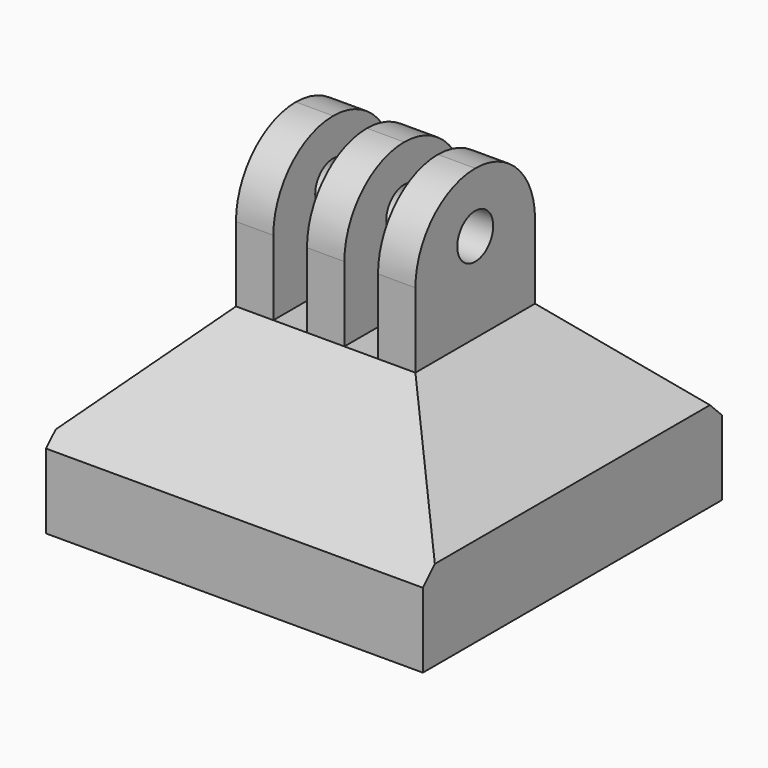
from build123d import *

# Parameters (mm, degrees)
F1_DEPTH     = 10
F2_R         = 4.99999
F3_W         = 7.5
F3_H         = 5
F3_W_2       = 10
F4_DEPTH     = 25.2
F5_T1_DEPTH  = 12
F5_T6_DEPTH  = 10
F5_T11_DEPTH = 10
F5_T17_DEPTH = 29.2876224097
F5_T23_DEPTH = 31.2876224097
F5_T31_DEPTH = 29.2876224097
F5_T37_DEPTH = 31.2876224097
F5_T45_DEPTH = 29.2876224097
F5_T51_DEPTH = 31.2876224097
F5_T59_DEPTH = 31.2876224097
F5_T64_DEPTH = 29.2876224097
F6_R         = 1.5
F7_DEPTH     = 25


# Not quite as in the source:
# - a fillet or chamfer that OpenCascade refuses, or shapes differently, is made with other operations: its cross-section is extruded or revolved along the edge and cut away or added
# - a fillet or chamfer is up to 0.001 mm smaller than in the source, because OpenCascade refuses the exact size


with BuildPart() as f1:
    # F0 (on Front) → F1 (new body)
    with BuildSketch(Plane.XZ):
        Polygon((12.5, -2.5), (12.5, 2.5), (6, 2.5), (-6, 2.5), (-12.5, 2.5), (-12.5, -2.5), align=None)
        Polygon((-6, 2.5), (6, 2.5), (6, 10), (6, 20), (3.5, 20), (3.5, 10), (1.25, 10), (1.25, 20), (0, 20), (-1.25, 20), (-1.25, 10), (-3.5, 10), (-3.5, 20), (-6, 20), (-6, 10), align=None)
    extrude(amount=F1_DEPTH)

    # F2 (radius 5 in the source; OpenCascade refuses exactly that, so slightly less here)
    f2_edges = [f1.edges().sort_by_distance(p)[0] for p in [
        (-4.75, 0, 20),
        (0, 0, 20),
        (4.75, 0, 20),
        (-4.75, -10, 20),
        (0, -10, 20),
        (4.75, -10, 20),
    ]]
    fillet(f2_edges, radius=F2_R)

    # F3 (on face) → F4 (join)
    with BuildSketch(Plane.YZ.offset(12.5)):
        with Locations((-13.75, 0)):
            Rectangle(F3_W, F3_H)
        with Locations((3.75, 0)):
            Rectangle(F3_W, F3_H)
        with Locations((-5, 0)):
            Rectangle(F3_W_2, F3_H)
    extrude(amount=-F4_DEPTH)

    # F5: chamfer of 7.5 on 4 edges, made by hand

    # F5_s2 → F5_t1 (join)
    with BuildSketch(Plane.YZ.offset(-6)):
        Polygon((-17.5, 2.5), (-10, 10), (-10, 2.5), align=None)
        Polygon((7.5, 2.5), (0, 10), (0, 2.5), align=None)
    extrude(amount=F5_T1_DEPTH)


with BuildPart() as f5_tool4:
    # F5_s5 → F5_t6 (new body)
    with BuildSketch(Plane.XZ):
        Polygon((6, 10), (13.5, 2.5), (6, 2.5), align=None)
    extrude(amount=F5_T6_DEPTH)

    split(bisect_by=Plane.YZ.offset(12.5), keep=Keep.BOTTOM)


with BuildPart() as f1_1:
    add(f1.part)

    # F5_t3: union F5_tool4
    add(f5_tool4.part)


with BuildPart() as f5_tool9:
    # F5_s10 → F5_t11 (new body)
    with BuildSketch(Plane.XZ):
        Polygon((-13.5, 2.5), (-6, 10), (-6, 2.5), align=None)
    extrude(amount=F5_T11_DEPTH)

    split(bisect_by=Plane.YZ.offset(-12.7), keep=Keep.TOP)


with BuildPart() as f1_2:
    add(f1_1.part)

    # F5_t8: union F5_tool9
    add(f5_tool9.part)


with BuildPart() as f5_tool15:
    # F5_s16 → F5_t17 (new body)
    with BuildSketch(Plane.XZ):
        Polygon((6, 10), (13.5, 2.5), (6, 2.5), align=None)
    extrude(amount=F5_T17_DEPTH)

    split(bisect_by=Plane.XZ.offset(17.5), keep=Keep.BOTTOM)

    split(bisect_by=Plane.YZ.offset(12.5), keep=Keep.BOTTOM)

    split(bisect_by=Plane.XZ.offset(10), keep=Keep.TOP)


with BuildPart() as f5_tool21:
    # F5_s22 → F5_t23 (new body)
    with BuildSketch(Plane.YZ.offset(25.2876224097)):
        Polygon((-17.5, 2.5), (-10, 10), (-10, 2.5), align=None)
    extrude(amount=-F5_T23_DEPTH)

    split(bisect_by=Plane.YZ.offset(6), keep=Keep.TOP)

    split(bisect_by=Plane.YZ.offset(12.5), keep=Keep.BOTTOM)


with BuildPart() as f5_tool15_1:
    add(f5_tool15.part)

    # F5_t26: intersect F5_tool21
    add(f5_tool21.part, mode=Mode.INTERSECT)


with BuildPart() as f1_3:
    add(f1_2.part)

    # F5_t13: union F5_tool15
    add(f5_tool15_1.part)


with BuildPart() as f5_tool29:
    # F5_s30 → F5_t31 (new body)
    with BuildSketch(Plane.XZ):
        Polygon((-13.5, 2.5), (-6, 10), (-6, 2.5), align=None)
    extrude(amount=F5_T31_DEPTH)

    split(bisect_by=Plane.YZ.offset(-12.7), keep=Keep.TOP)

    split(bisect_by=Plane.XZ.offset(17.5), keep=Keep.BOTTOM)

    split(bisect_by=Plane.XZ.offset(10), keep=Keep.TOP)


with BuildPart() as f5_tool35:
    # F5_s36 → F5_t37 (new body)
    with BuildSketch(Plane.YZ.offset(6)):
        Polygon((-17.5, 2.5), (-10, 10), (-10, 2.5), align=None)
    extrude(amount=-F5_T37_DEPTH)

    split(bisect_by=Plane.YZ.offset(-6), keep=Keep.BOTTOM)

    split(bisect_by=Plane.YZ.offset(-12.7), keep=Keep.TOP)


with BuildPart() as f5_tool29_1:
    add(f5_tool29.part)

    # F5_t40: intersect F5_tool35
    add(f5_tool35.part, mode=Mode.INTERSECT)


with BuildPart() as f1_4:
    add(f1_3.part)

    # F5_t27: union F5_tool29
    add(f5_tool29_1.part)


with BuildPart() as f5_tool43:
    # F5_s44 → F5_t45 (new body)
    with BuildSketch(Plane.XZ.offset(-19.2876224097)):
        Polygon((6, 10), (13.5, 2.5), (6, 2.5), align=None)
    extrude(amount=F5_T45_DEPTH)

    split(bisect_by=Plane.XZ.offset(-7.5), keep=Keep.TOP)

    split(bisect_by=Plane.YZ.offset(12.5), keep=Keep.BOTTOM)

    split(bisect_by=Plane.XZ, keep=Keep.BOTTOM)


with BuildPart() as f5_tool49:
    # F5_s50 → F5_t51 (new body)
    with BuildSketch(Plane.YZ.offset(25.2876224097)):
        Polygon((7.5, 2.5), (0, 10), (0, 2.5), align=None)
    extrude(amount=-F5_T51_DEPTH)

    split(bisect_by=Plane.YZ.offset(6), keep=Keep.TOP)

    split(bisect_by=Plane.YZ.offset(12.5), keep=Keep.BOTTOM)


with BuildPart() as f5_tool43_1:
    add(f5_tool43.part)

    # F5_t54: intersect F5_tool49
    add(f5_tool49.part, mode=Mode.INTERSECT)


with BuildPart() as f1_5:
    add(f1_4.part)

    # F5_t41: union F5_tool43
    add(f5_tool43_1.part)


with BuildPart() as f5_tool57:
    # F5_s58 → F5_t59 (new body)
    with BuildSketch(Plane.YZ.offset(6)):
        Polygon((7.5, 2.5), (0, 10), (0, 2.5), align=None)
    extrude(amount=-F5_T59_DEPTH)

    split(bisect_by=Plane.YZ.offset(-6), keep=Keep.BOTTOM)

    split(bisect_by=Plane.YZ.offset(-12.7), keep=Keep.TOP)


with BuildPart() as f5_tool62:
    # F5_s63 → F5_t64 (new body)
    with BuildSketch(Plane.XZ.offset(-19.2876224097)):
        Polygon((-13.5, 2.5), (-6, 10), (-6, 2.5), align=None)
    extrude(amount=F5_T64_DEPTH)

    split(bisect_by=Plane.XZ.offset(-7.5), keep=Keep.TOP)

    split(bisect_by=Plane.YZ.offset(-12.7), keep=Keep.TOP)

    split(bisect_by=Plane.XZ, keep=Keep.BOTTOM)


with BuildPart() as f5_tool57_1:
    add(f5_tool57.part)

    # F5_t68: intersect F5_tool62
    add(f5_tool62.part, mode=Mode.INTERSECT)


with BuildPart() as f1_6:
    add(f1_5.part)

    # F5_t55: union F5_tool57
    add(f5_tool57_1.part)

    # F6 (on face) → F7 (cut)
    with BuildSketch(Plane(origin=(-6, 0, 0), x_dir=(0, -1, 0), z_dir=(-1, 0, 0))):
        with Locations((5, 16)):
            Circle(F6_R)
    extrude(amount=-F7_DEPTH, mode=Mode.SUBTRACT)


solid = f1_6.part
